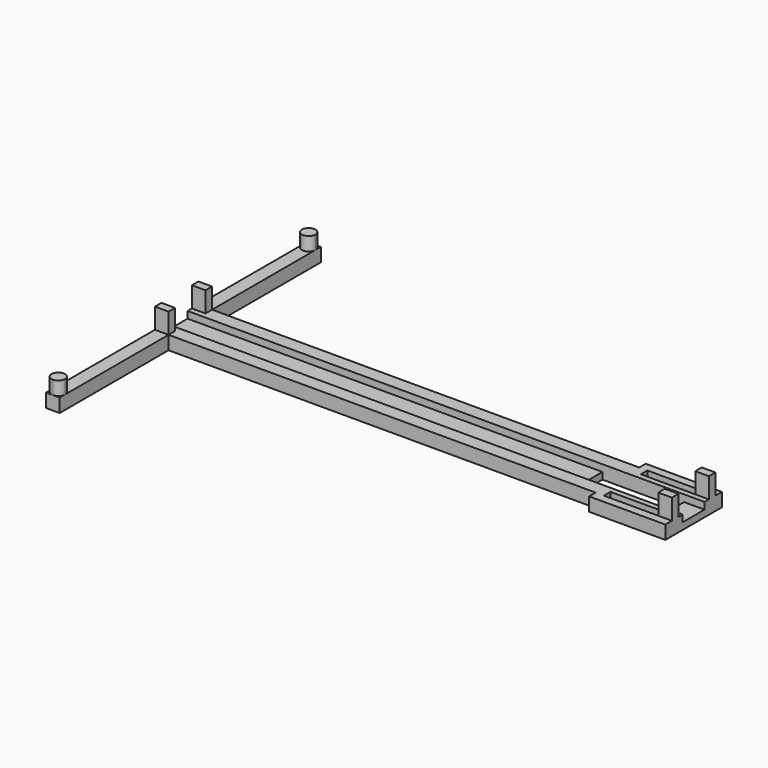
from build123d import *

# Parameters (mm, degrees)
F1_DEPTH  = 5
F2_W      = 10
F2_H      = 2.5
F3_DEPTH  = 200
F4_W      = 5
F4_H      = 3
F5_DEPTH  = 7.5
F6_W      = 5
F6_H      = 5
F7_DEPTH  = 50
F8_W      = 5
F8_H      = 5
F9_DEPTH  = 50
F12_DEPTH = 5


# Not quite as in the source:
# - a feature names something its author has since deleted; it is built from what else it names


with BuildPart() as f1:
    # F0 (on Top) → F1 (new body)
    with BuildSketch(Plane.XY):
        Polygon((-100, 10), (-100, 0), (-100, -10), (62, -10), (65, -10), (65, -7), (85, -7), (85, -10), (90, -10), (90, 0), (90, 10), (85, 10), (85, 7), (65, 7), (65, 10), (62, 10), align=None)
        Polygon((82.5, 5), (82.5, 0), (82.5, -5), (52.5, -5), (52.5, 0), (52.5, 5), align=None, mode=Mode.SUBTRACT)
        Polygon((65, -10), (62, -10), (62, -13), (90, -13), (90, -10), (85, -10), align=None)
        Polygon((62, 13), (62, 10), (65, 10), (85, 10), (90, 10), (90, 13), align=None)
    extrude(amount=F1_DEPTH)

    # F2 (on face) → F3 (cut)
    with BuildSketch(Plane.YZ.offset(90)):
        with Locations((0, 3.75)):
            Rectangle(F2_W, F2_H)
    extrude(amount=-F3_DEPTH, mode=Mode.SUBTRACT)

    # F4 (on face) → F5 (join)
    with BuildSketch(Plane.XY.offset(5)):
        with Locations((-97.5, 8.5)):
            Rectangle(F4_W, F4_H)
        with Locations((-97.5, -8.5)):
            Rectangle(F4_W, F4_H)
        with Locations((87.5, -8.5)):
            Rectangle(F4_W, F4_H)
        with Locations((87.5, 8.5)):
            Rectangle(F4_W, F4_H)
    extrude(amount=F5_DEPTH)

    # F6 (on face) → F7 (join)
    with BuildSketch(Plane.XZ.offset(10)):
        with Locations((-97.5, 2.5)):
            Rectangle(F6_W, F6_H)
    extrude(amount=F7_DEPTH)

    # F8 (on face) → F9 (join)
    with BuildSketch(Plane(origin=(0, 10, 0), x_dir=(-1, 0, 0), z_dir=(0, 1, 0))):
        with Locations((97.5, 2.5)):
            Rectangle(F8_W, F8_H)
    extrude(amount=F9_DEPTH)

    # F10 (on face) + F11 (on face) → F12 (join)
    with BuildSketch(Plane.XY.offset(5)):
        with BuildLine():
            ThreePointArc((-100, -57.5), (-99.267766953, -59.267766953), (-97.5, -60))
            ThreePointArc((-97.5, -60), (-95.732233047, -59.267766953), (-95, -57.5))
            ThreePointArc((-95, -57.5), (-97.5, -55), (-100, -57.5))
        make_face()
    with BuildSketch(Plane.XY.offset(5)):
        with BuildLine():
            ThreePointArc((-100, 57.5), (-97.5, 55), (-95, 57.5))
            ThreePointArc((-95, 57.5), (-95.732233047, 59.267766953), (-97.5, 60))
            ThreePointArc((-97.5, 60), (-99.267766953, 59.267766953), (-100, 57.5))
        make_face()
    extrude(amount=F12_DEPTH)


solid = f1.part
